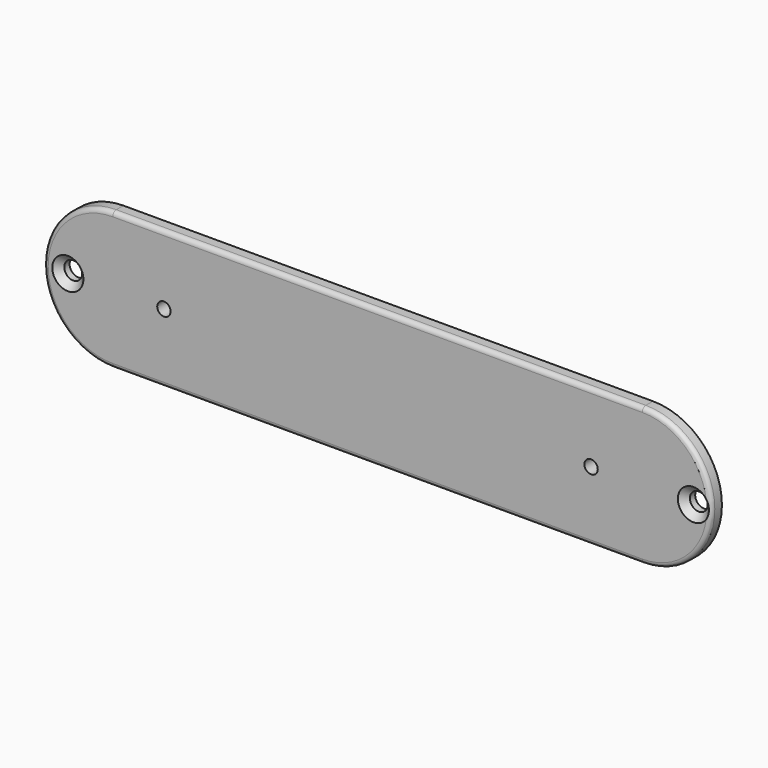
from build123d import *

# Parameters (mm, degrees)
F0_R     = 2
F0_R_2   = 1.5
F1_DEPTH = 3
F2_R     = 1


# Not quite as in the source:
# - a fillet or chamfer that OpenCascade refuses, or shapes differently, is made with other operations: its cross-section is extruded or revolved along the edge and cut away or added


with BuildPart() as f1:
    # F0 (on Front) → F1 (new body)
    with BuildSketch(Plane.XZ):
        with BuildLine():
            Line((59.5, 15.5), (-59.5, 15.5))
            ThreePointArc((-59.5, 15.5), (-75, 0), (-59.5, -15.5))
            Line((-59.5, -15.5), (59.5, -15.5))
            ThreePointArc((59.5, -15.5), (75, 0), (59.5, 15.5))
        make_face()
        with Locations((-69.59, 0)):
            Circle(F0_R, mode=Mode.SUBTRACT)
        with Locations((-48, 0)):
            Circle(F0_R_2, mode=Mode.SUBTRACT)
        with Locations((48, 0)):
            Circle(F0_R_2, mode=Mode.SUBTRACT)
        with Locations((71, 0)):
            Circle(F0_R, mode=Mode.SUBTRACT)
    extrude(amount=F1_DEPTH)

    # F2
    f2_edges = [f1.edges().sort_by_distance(p)[0] for p in [
        (0, -3, 15.5),
        (-75, -3, 0),
        (0, -3, -15.5),
        (75, -3, 0),
    ]]
    fillet(f2_edges, radius=F2_R)

    # F3: chamfer of 1.5 on 2 edges, made by hand

    # F3_s1 → F3_t2 (revolve, cut)
    with BuildSketch(Plane.XY):
        Polygon((-66.09, -3), (-67.59, -1.5), (-67.59, -3), align=None)
    revolve(axis=Axis((-69.59, -3, 0), (0, -1, 0)), mode=Mode.SUBTRACT)

    # F3_s3 → F3_t4 (revolve, cut)
    with BuildSketch(Plane.XY):
        Polygon((74.5, -3), (73, -1.5), (73, -3), align=None)
    revolve(axis=Axis((71, -3, 0), (0, -1, 0)), mode=Mode.SUBTRACT)


solid = f1.part
